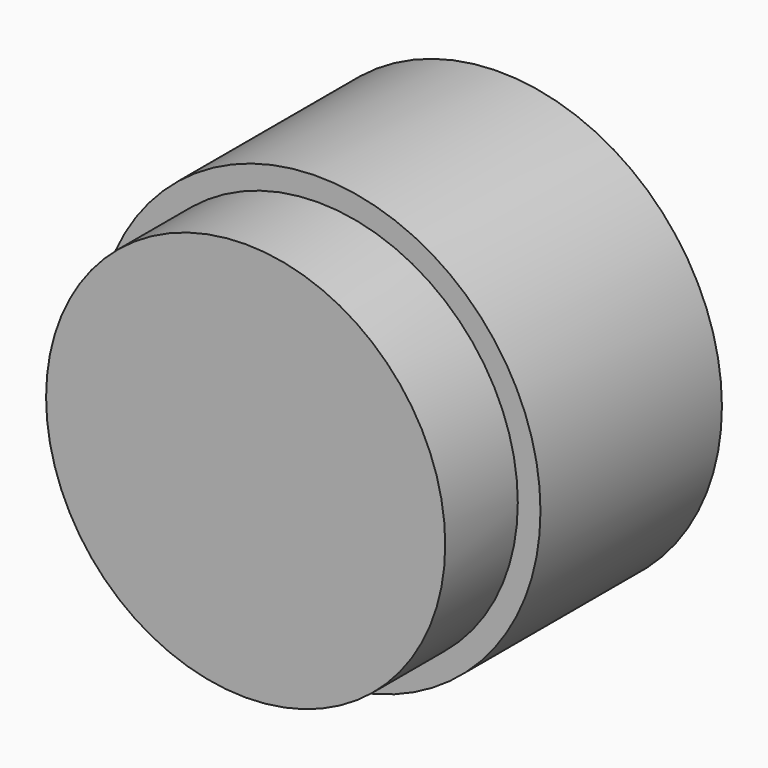
from build123d import *

# Parameters (mm, degrees)
F0_R     = 22
F2_DEPTH = 25
F3_DEPTH = 25
F4_R     = 24.5
F5_DEPTH = 25


with BuildPart() as f2:
    # F0 (on Front) → F2 (new body)
    with BuildSketch(Plane.XZ):
        Circle(F0_R)
        with BuildLine():
            ThreePointArc((-19.401899791, 1.9535312895), (-13.921825835, 13.654038429), (-2.3299484959, 19.3603032003))
            ThreePointArc((-2.3299484959, 19.3603032003), (0, 19.5), (2.3299484959, 19.3603032003))
            ThreePointArc((2.3299484959, 19.3603032003), (13.921825835, 13.654038429), (19.401899791, 1.9535312895))
            ThreePointArc((19.401899791, 1.9535312895), (19.4754595058, 0.9779964404), (19.5, 0))
            ThreePointArc((19.5, 0), (19.4754595058, -0.9779964404), (19.401899791, -1.9535312895))
            ThreePointArc((19.401899791, -1.9535312895), (13.921825835, -13.654038429), (2.3299484959, -19.3603032003))
            ThreePointArc((2.3299484959, -19.3603032003), (0, -19.5), (-2.3299484959, -19.3603032003))
            ThreePointArc((-2.3299484959, -19.3603032003), (-13.921825835, -13.654038429), (-19.401899791, -1.9535312895))
            ThreePointArc((-19.401899791, -1.9535312895), (-19.5, 0), (-19.401899791, 1.9535312895))
        make_face(mode=Mode.SUBTRACT)
    extrude(amount=F2_DEPTH)



with BuildPart() as f2b:
    # F0 (on Front) → F2, piece 2 (new body)
    with BuildSketch(Plane.XZ):
        with BuildLine():
            ThreePointArc((-2.8938206378, 1.9535312895), (-1.7519205381, 1.9616594322), (-1.1833040417, 2.9519508966))
            ThreePointArc((-1.1833040417, 2.9519508966), (-1.5191484267, 3.7627509657), (-2.3299484959, 4.0985953507))
            ThreePointArc((-2.3299484959, 4.0985953507), (-3.4389177943, 3.2434652177), (-2.8938206378, 1.9535312895))
        make_face()
    extrude(amount=F2_DEPTH)


with BuildPart() as f2_1:
    add(f2.part)

    add(f2b.part)  # F3 merges F2b
    # F0 (on Front) → F3 (join)
    with BuildSketch(Plane.XZ):
        with BuildLine():
            ThreePointArc((-2.8938206378, 1.9535312895), (-3.4389177943, 3.2434652177), (-2.3299484959, 4.0985953507))
            Line((-2.3299484959, 4.0985953507), (-2.3299484959, 19.3603032003))
            ThreePointArc((-2.3299484959, 19.3603032003), (-13.921825835, 13.654038429), (-19.401899791, 1.9535312895))
            Line((-19.401899791, 1.9535312895), (-2.8938206378, 1.9535312895))
        make_face()
        with BuildLine():
            ThreePointArc((19.401899791, 1.9535312895), (13.921825835, 13.654038429), (2.3299484959, 19.3603032003))
            Line((2.3299484959, 19.3603032003), (2.3299484959, 4.0985953507))
            ThreePointArc((2.3299484959, 4.0985953507), (3.140748565, 3.7627509657), (3.47659295, 2.9519508966))
            ThreePointArc((3.47659295, 2.9519508966), (3.3202399602, 2.3739229388), (2.8938206378, 1.9535312895))
            Line((2.8938206378, 1.9535312895), (19.401899791, 1.9535312895))
        make_face()
        with BuildLine():
            ThreePointArc((-2.3299484959, 4.0985953507), (-1.5191484267, 3.7627509657), (-1.1833040417, 2.9519508966))
            ThreePointArc((-1.1833040417, 2.9519508966), (-1.7519205381, 1.9616594322), (-2.8938206378, 1.9535312895))
            Line((-2.8938206378, 1.9535312895), (-19.401899791, 1.9535312895))
            ThreePointArc((-19.401899791, 1.9535312895), (-19.5, 0), (-19.401899791, -1.9535312895))
            Line((-19.401899791, -1.9535312895), (-2.8938206378, -1.9535312895))
            ThreePointArc((-2.8938206378, -1.9535312895), (-1.7519205381, -1.9616594322), (-1.1833040417, -2.9519508966))
            ThreePointArc((-1.1833040417, -2.9519508966), (-1.5191484267, -3.7627509657), (-2.3299484959, -4.0985953507))
            Line((-2.3299484959, -4.0985953507), (-2.3299484959, -19.3603032003))
            ThreePointArc((-2.3299484959, -19.3603032003), (0, -19.5), (2.3299484959, -19.3603032003))
            Line((2.3299484959, -19.3603032003), (2.3299484959, -4.0985953507))
            ThreePointArc((2.3299484959, -4.0985953507), (1.2209791974, -2.6604365754), (2.8938206378, -1.9535312895))
            Line((2.8938206378, -1.9535312895), (19.401899791, -1.9535312895))
            ThreePointArc((19.401899791, -1.9535312895), (19.4754595058, -0.9779964404), (19.5, 0))
            ThreePointArc((19.5, 0), (19.4754595058, 0.9779964404), (19.401899791, 1.9535312895))
            Line((19.401899791, 1.9535312895), (2.8938206378, 1.9535312895))
            ThreePointArc((2.8938206378, 1.9535312895), (1.2209791974, 2.6604365754), (2.3299484959, 4.0985953507))
            Line((2.3299484959, 4.0985953507), (2.3299484959, 19.3603032003))
            ThreePointArc((2.3299484959, 19.3603032003), (0, 19.5), (-2.3299484959, 19.3603032003))
            Line((-2.3299484959, 19.3603032003), (-2.3299484959, 4.0985953507))
        make_face()
        with BuildLine():
            Line((-2.8938206378, -1.9535312895), (-19.401899791, -1.9535312895))
            ThreePointArc((-19.401899791, -1.9535312895), (-13.921825835, -13.654038429), (-2.3299484959, -19.3603032003))
            Line((-2.3299484959, -19.3603032003), (-2.3299484959, -4.0985953507))
            ThreePointArc((-2.3299484959, -4.0985953507), (-3.4389177943, -3.2434652177), (-2.8938206378, -1.9535312895))
        make_face()
        with BuildLine():
            Line((2.3299484959, -4.0985953507), (2.3299484959, -19.3603032003))
            ThreePointArc((2.3299484959, -19.3603032003), (13.921825835, -13.654038429), (19.401899791, -1.9535312895))
            Line((19.401899791, -1.9535312895), (2.8938206378, -1.9535312895))
            ThreePointArc((2.8938206378, -1.9535312895), (3.3202399602, -2.3739229388), (3.47659295, -2.9519508966))
            ThreePointArc((3.47659295, -2.9519508966), (3.140748565, -3.7627509657), (2.3299484959, -4.0985953507))
        make_face()
        with BuildLine():
            ThreePointArc((2.8938206378, -1.9535312895), (1.2209791974, -2.6604365754), (2.3299484959, -4.0985953507))
            ThreePointArc((2.3299484959, -4.0985953507), (3.140748565, -3.7627509657), (3.47659295, -2.9519508966))
            ThreePointArc((3.47659295, -2.9519508966), (3.3202399602, -2.3739229388), (2.8938206378, -1.9535312895))
        make_face()
        with BuildLine():
            ThreePointArc((3.47659295, 2.9519508966), (3.140748565, 3.7627509657), (2.3299484959, 4.0985953507))
            ThreePointArc((2.3299484959, 4.0985953507), (1.2209791974, 2.6604365754), (2.8938206378, 1.9535312895))
            ThreePointArc((2.8938206378, 1.9535312895), (3.3202399602, 2.3739229388), (3.47659295, 2.9519508966))
        make_face()
        with BuildLine():
            ThreePointArc((-1.1833040417, -2.9519508966), (-1.7519205381, -1.9616594322), (-2.8938206378, -1.9535312895))
            ThreePointArc((-2.8938206378, -1.9535312895), (-3.4389177943, -3.2434652177), (-2.3299484959, -4.0985953507))
            ThreePointArc((-2.3299484959, -4.0985953507), (-1.5191484267, -3.7627509657), (-1.1833040417, -2.9519508966))
        make_face()
    extrude(amount=F3_DEPTH)

    # F4 (on offset) → F5 (join)
    with BuildSketch(Plane.XZ.offset(15)):
        Circle(F4_R)
    extrude(amount=-F5_DEPTH)


solid = f2_1.part
